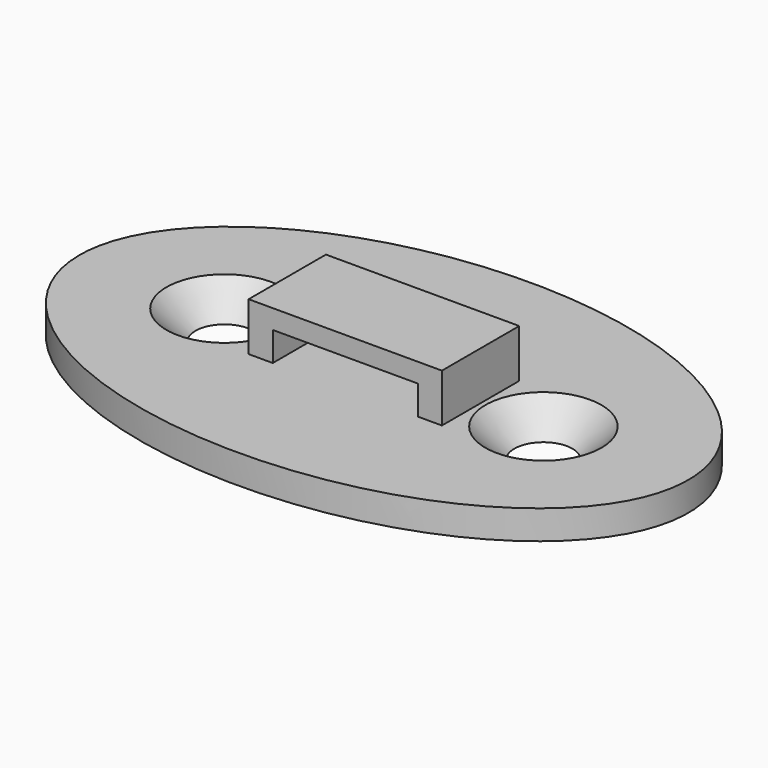
from build123d import *

# Parameters (mm, degrees)
F0_R     = 3
F1_DEPTH = 3
F3_DEPTH = 5
F4_SIZE  = 2.99999


# Not quite as in the source:
# - a fillet or chamfer is up to 0.001 mm smaller than in the source, because OpenCascade refuses the exact size


with BuildPart() as f1:
    # F0 (on Top) → F1 (new body)
    with BuildSketch(Plane.XY):
        with BuildLine():
            add(Edge.make_bspline(
                [(-31.5, 0), (-31.5, -32.9089653438), (15.75, -16.4544826719), (63, 0), (15.75, 16.4544826719), (-31.5, 32.9089653438), (-31.5, 0)],
                knots=[0, 0, 0, 2.0943951024, 2.0943951024, 4.1887902048, 4.1887902048, 6.2831853072, 6.2831853072, 6.2831853072], degree=2, weights=[1, 0.5, 1, 0.5, 1, 0.5, 1]))
        make_face()
        with Locations((-16.5, 0)):
            Circle(F0_R, mode=Mode.SUBTRACT)
        with Locations((16.5, 0)):
            Circle(F0_R, mode=Mode.SUBTRACT)
    extrude(amount=F1_DEPTH)

    # F2 (on Front) → F3 (join, symmetric)
    with BuildSketch(Plane.XZ):
        Polygon((7.5, 3), (10, 3), (10, 8), (-10, 8), (-10, 3), (-7.5, 3), (-7.5, 6.0126003809), (7.5, 6.0126003809), align=None)
    extrude(amount=F3_DEPTH, both=True)

    # F4 (size 3 in the source; OpenCascade refuses exactly that, so slightly less here)
    f4_edges = [f1.edges().sort_by_distance(p)[0] for p in [
        (-19.5, 0, 3),
        (13.5, 0, 3),
    ]]
    chamfer(f4_edges, length=F4_SIZE)


solid = f1.part
